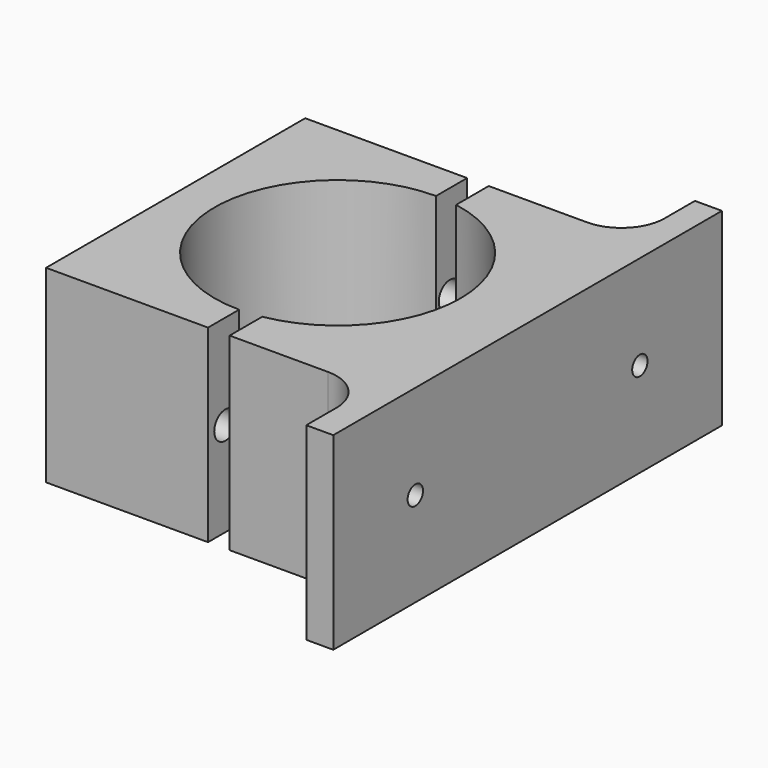
from build123d import *

# Parameters (mm, degrees)
F1_DEPTH = 22.225
F2_R     = 1.1303
F3_DEPTH = 41.403
F4_R     = 5.08
F5_R     = 1.6256
F6_DEPTH = 41.403


with BuildPart() as f1:
    # F0 (on Top) → F1 (new body)
    with BuildSketch(Plane.XY):
        with BuildLine():
            Line((-9.906, -19.05), (6.731, -19.05))
            Line((6.731, -19.05), (6.731, -28.575))
            Line((6.731, -28.575), (9.906, -28.575))
            Line((9.906, -28.575), (9.906, -19.05))
            Line((9.906, -19.05), (9.906, 19.05))
            Line((9.906, 19.05), (9.906, 28.575))
            Line((9.906, 28.575), (6.731, 28.575))
            Line((6.731, 28.575), (6.731, 19.05))
            Line((6.731, 19.05), (-9.906, 19.05))
            Line((-9.906, 19.05), (-9.906, 14.2534516521))
            ThreePointArc((-9.906, 14.2534516521), (2.032, 0), (-9.906, -14.2534516521))
            Line((-9.906, -14.2534516521), (-9.906, -19.05))
        make_face()
    extrude(amount=F1_DEPTH)


with BuildPart() as f1b:
    # F0 (on Top) → F1, piece 2 (new body)
    with BuildSketch(Plane.XY):
        with BuildLine():
            ThreePointArc((-12.446, -14.478), (-26.924, 0), (-12.446, 14.478))
            Line((-12.446, 14.478), (-12.446, 19.05))
            Line((-12.446, 19.05), (-31.496, 19.05))
            Line((-31.496, 19.05), (-31.496, -19.05))
            Line((-31.496, -19.05), (-12.446, -19.05))
            Line((-12.446, -19.05), (-12.446, -14.478))
        make_face()
    extrude(amount=F1_DEPTH)


with BuildPart() as f3_tool:
    # F2 (on face) → F3 (new body, through all)
    with BuildSketch(Plane.YZ.offset(9.906)):
        with Locations((16.51, 11.1125)):
            Circle(F2_R)
        with Locations((-16.51, 11.1125)):
            Circle(F2_R)
    extrude(amount=-F3_DEPTH)


with BuildPart() as f1_1:
    add(f1.part)

    # F3: cut by f3_tool
    add(f3_tool.part, mode=Mode.SUBTRACT)

    # F4
    f4_edges = [f1_1.edges().sort_by_distance(p)[0] for p in [
        (6.731, -19.05, 11.1125),
        (6.731, 19.05, 11.1125),
    ]]
    fillet(f4_edges, radius=F4_R)


with BuildPart() as f1b_1:
    add(f1b.part)

    # F3: cut by f3_tool
    add(f3_tool.part, mode=Mode.SUBTRACT)

    # F5 (on face) → F6 (cut, through all)
    with BuildSketch(Plane(origin=(-31.496, 0, 0), x_dir=(0, -1, 0), z_dir=(-1, 0, 0))):
        with Locations((16.51, 11.0998)):
            Circle(F5_R)
        with Locations((-16.51, 11.0998)):
            Circle(F5_R)
    extrude(amount=-F6_DEPTH, mode=Mode.SUBTRACT)


solid = Compound([f1_1.part, f1b_1.part])
